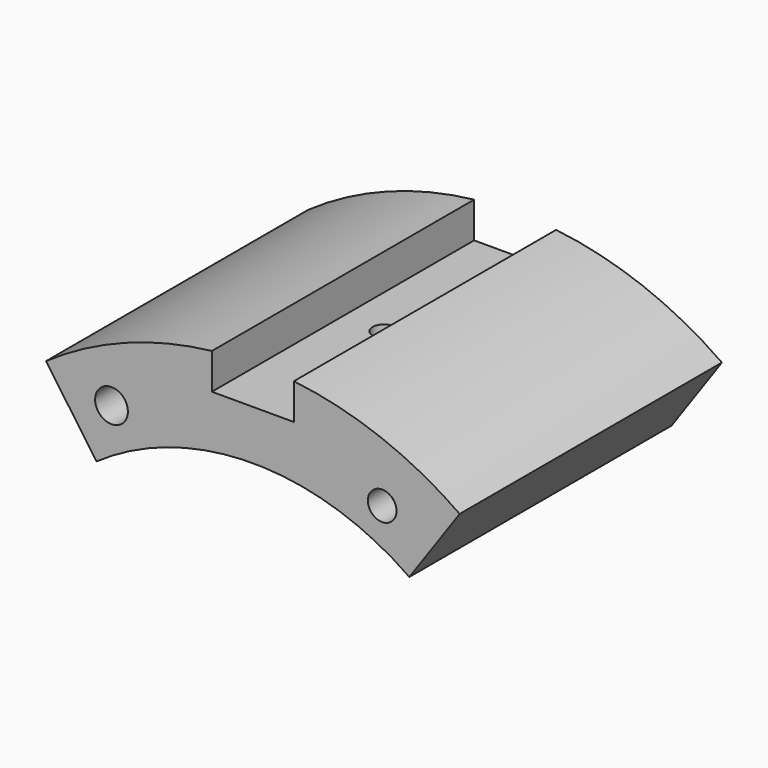
from build123d import *

# Parameters (mm, degrees)
F3_DEPTH  = 60
F9_D      = 6
F9_DEPTH  = 35
F9_TIP    = 1.8025818571
F10_D     = 4.2
F10_DEPTH = 4.8
F10_TIP   = 1.2618073
F11_DEPTH = 12
F12_D     = 5.25


# Not quite as in the source:
# - a feature of the source that left no trace in its solid (it failed there, or was rolled back) is left out
# - a feature names something its author has since deleted; it is built from what else it names


with BuildPart() as f3:
    # F2 (on Front) → F3 (new body)
    with BuildSketch(Plane.XZ):
        with BuildLine():
            ThreePointArc((-28.634656432, 40.894527507), (0, 49.923), (28.634656432, 40.894527507))
            Line((28.634656432, 40.894527507), (37.8560447992, 54.0640349231))
            ThreePointArc((37.8560447992, 54.0640349231), (23.3966615381, 61.7138252653), (7.5, 65.5724789832))
            Line((7.5, 65.5724789832), (7.5, 59))
            Line((7.5, 59), (0, 59))
            Line((0, 59), (-7.5, 59))
            Line((-7.5, 59), (-7.5, 65.5724789832))
            ThreePointArc((-7.5, 65.5724789832), (-23.3966615381, 61.7138252653), (-37.8560447992, 54.0640349231))
            Line((-37.8560447992, 54.0640349231), (-28.634656432, 40.894527507))
        make_face()
    extrude(amount=F3_DEPTH)

    # F9
    with Locations(Plane.XZ.offset(60)):
        with Locations((-25.8774584852, 50.7873718787)):
            Hole(F9_D / 2, depth=F9_DEPTH)
            with Locations((0, 0, -(F9_DEPTH + F9_TIP / 2))):  # 118° drill point
                Cone(0, F9_D / 2, F9_TIP, mode=Mode.SUBTRACT)

    # F10
    with Locations(Plane.XY.offset(59)):
        with Locations((0, -30)):
            Hole(F10_D / 2, depth=F10_DEPTH)
            with Locations((0, 0, -(F10_DEPTH + F10_TIP / 2))):  # 118° drill point
                Cone(0, F10_D / 2, F10_TIP, mode=Mode.SUBTRACT)

    # F7 (on line) → F11 (cut)
    with BuildSketch(Plane(origin=(21.0180858076, 0, 45.0734304703), x_dir=(0.906307787, 0, -0.4226182617), z_dir=(0.4226182617, 0, 0.906307787))):
        with BuildLine():
            Line((0, -5), (0, -55))
            Line((0, -55), (3.487631816, -55))
            ThreePointArc((3.487631816, -55), (4.1947385971, -54.7071067812), (4.487631816, -54))
            Line((4.487631816, -54), (4.487631816, -6))
            ThreePointArc((4.487631816, -6), (4.1947385971, -5.2928932188), (3.487631816, -5))
            Line((3.487631816, -5), (0, -5))
        make_face()
        with BuildLine():
            Line((-3.359387327, -55), (0, -55))
            Line((0, -55), (0, -5))
            Line((0, -5), (-3.359387327, -5))
            ThreePointArc((-3.359387327, -5), (-4.0664941082, -5.2928932188), (-4.359387327, -6))
            Line((-4.359387327, -6), (-4.359387327, -54))
            ThreePointArc((-4.359387327, -54), (-4.0664941082, -54.7071067812), (-3.359387327, -55))
        make_face()
    extrude(amount=F11_DEPTH, mode=Mode.SUBTRACT)

    # F12 (through all)
    with Locations(Plane.XZ.offset(60)):
        with Locations((23.6666226575, 50.7532360741)):
            Hole(F12_D / 2)


solid = f3.part
